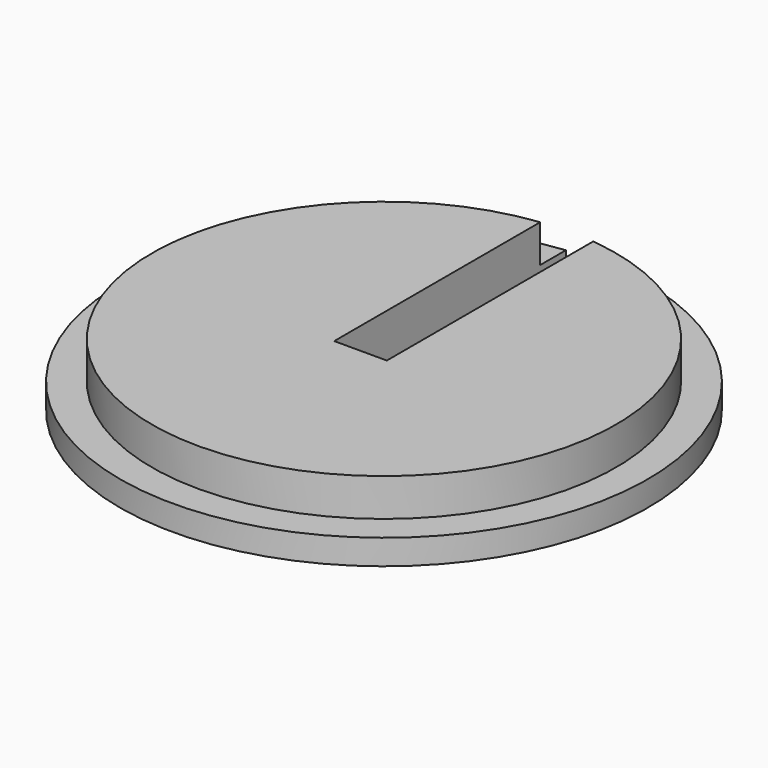
from build123d import *

# Parameters (mm, degrees)
F0_R         = 31.5
F1_DEPTH     = 3
F2_R         = 27.7
F3_DEPTH     = 4.5
F4_W         = 6.2837838195
F4_H         = 36.2837854773
F5_DEPTH     = 25
F6_TEXT_SIZE = 6.9512805962
F7_DEPTH     = 1.5


# Not quite as in the source:
# - Text() gives the source's letters only with a copy of the font that has no kerning and outlines rounded to 1/6400 em; it was checked with that copy


with BuildPart() as f1:
    # F0 (on Top) → F1 (new body)
    with BuildSketch(Plane.XY):
        Circle(F0_R)
    extrude(amount=F1_DEPTH)

    # F2 (on face) → F3 (join)
    with BuildSketch(Plane.XY.offset(3)):
        Circle(F2_R)
    extrude(amount=F3_DEPTH)

    # F4 (on face) → F5 (cut)
    with BuildSketch(Plane(origin=(0, 0, 0), x_dir=(1, 0, 0), z_dir=(0, 0, -1))):
        with Locations((-0.2027030569, -14.8986494169)):
            Rectangle(F4_W, F4_H)
    extrude(amount=-F5_DEPTH, mode=Mode.SUBTRACT)

    # F6 (on face) → F7 (cut)
    with BuildSketch(Plane(origin=(0, 0, 0), x_dir=(1, 0, 0), z_dir=(0, 0, -1))):
        with Locations((-26.4974127228, 7.6181068004)):
            Text('757 Makerspace', F6_TEXT_SIZE, font='Open Sans', text_align=(TextAlign.LEFT, TextAlign.BOTTOM))
    extrude(amount=-F7_DEPTH, mode=Mode.SUBTRACT)


solid = f1.part
